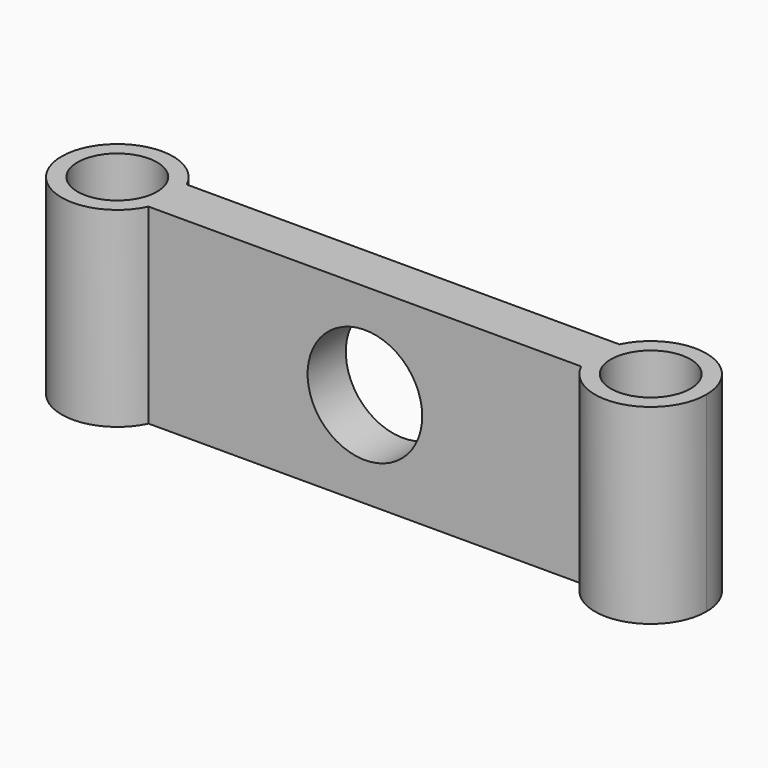
from build123d import *

# Parameters (mm, degrees)
F1_DEPTH = 12
F2_D     = 5
F2_DEPTH = 15
F2_TIP   = 1.5021515476
F3_D     = 5
F3_DEPTH = 15
F3_TIP   = 1.5021515476
F5_D     = 7.2
F5_DEPTH = 10
F5_TIP   = 2.1630982285


# Not quite as in the source:
# - a feature names something its author has since deleted; it is built from what else it names


with BuildPart() as f1:
    # F0 (on Top) → F1 (new body)
    with BuildSketch(Plane.XY):
        with BuildLine():
            Line((-14.5, -1.8754155822), (-14.5, 1.1245844178))
            Line((-14.5, 1.1245844178), (-11.3377223398, 1.1245844178))
            ThreePointArc((-11.3377223398, 1.1245844178), (-18, -0.3754155822), (-11.3377223398, -1.8754155822))
            Line((-11.3377223398, -1.8754155822), (-14.5, -1.8754155822))
        make_face()
        with BuildLine():
            Line((-11.3377223398, 1.1245844178), (-14.5, 1.1245844178))
            Line((-14.5, 1.1245844178), (-14.5, -1.8754155822))
            Line((-14.5, -1.8754155822), (-11.3377223398, -1.8754155822))
            ThreePointArc((-11.3377223398, -1.8754155822), (-11.0854742781, -1.144189993), (-11, -0.3754155822))
            ThreePointArc((-11, -0.3754155822), (-11.0854742781, 0.3933588286), (-11.3377223398, 1.1245844178))
        make_face()
        with BuildLine():
            Line((15.8377223398, 1.1245844178), (-11.3377223398, 1.1245844178))
            ThreePointArc((-11.3377223398, 1.1245844178), (-11.0854742781, 0.3933588286), (-11, -0.3754155822))
            ThreePointArc((-11, -0.3754155822), (-11.0854742781, -1.144189993), (-11.3377223398, -1.8754155822))
            Line((-11.3377223398, -1.8754155822), (15.8377223398, -1.8754155822))
            ThreePointArc((15.8377223398, -1.8754155822), (15.5, -0.3754155822), (15.8377223398, 1.1245844178))
        make_face()
        with BuildLine():
            ThreePointArc((22.5, -0.3754155822), (19.7687744108, 3.0391101397), (15.8377223398, 1.1245844178))
            Line((15.8377223398, 1.1245844178), (19, 1.1245844178))
            Line((19, 1.1245844178), (19, -1.8754155822))
            Line((19, -1.8754155822), (15.8377223398, -1.8754155822))
            ThreePointArc((15.8377223398, -1.8754155822), (19.7687744108, -3.7899413041), (22.5, -0.3754155822))
        make_face()
        with BuildLine():
            Line((19, 1.1245844178), (15.8377223398, 1.1245844178))
            ThreePointArc((15.8377223398, 1.1245844178), (15.5, -0.3754155822), (15.8377223398, -1.8754155822))
            Line((15.8377223398, -1.8754155822), (19, -1.8754155822))
            Line((19, -1.8754155822), (19, 1.1245844178))
        make_face()
    extrude(amount=F1_DEPTH)

    # F2
    with Locations(Plane(origin=(0, 0, 0), x_dir=(1, 0, 0), z_dir=(0, 0, -1))):
        with Locations((19, 0.3754155822)):
            Hole(F2_D / 2, depth=F2_DEPTH)
            with Locations((0, 0, -(F2_DEPTH + F2_TIP / 2))):  # 118° drill point
                Cone(0, F2_D / 2, F2_TIP, mode=Mode.SUBTRACT)

    # F3
    with Locations(Plane(origin=(0, 0, 0), x_dir=(1, 0, 0), z_dir=(0, 0, -1))):
        with Locations((-14.5, 0.3754155822)):
            Hole(F3_D / 2, depth=F3_DEPTH)
            with Locations((0, 0, -(F3_DEPTH + F3_TIP / 2))):  # 118° drill point
                Cone(0, F3_D / 2, F3_TIP, mode=Mode.SUBTRACT)

    # F5
    with Locations(Plane(origin=(0, 1.1245844178, 0), x_dir=(-1, 0, 0), z_dir=(0, 1, 0))):
        with Locations((-2.25, 6)):
            Hole(F5_D / 2, depth=F5_DEPTH)
            with Locations((0, 0, -(F5_DEPTH + F5_TIP / 2))):  # 118° drill point
                Cone(0, F5_D / 2, F5_TIP, mode=Mode.SUBTRACT)


solid = f1.part
